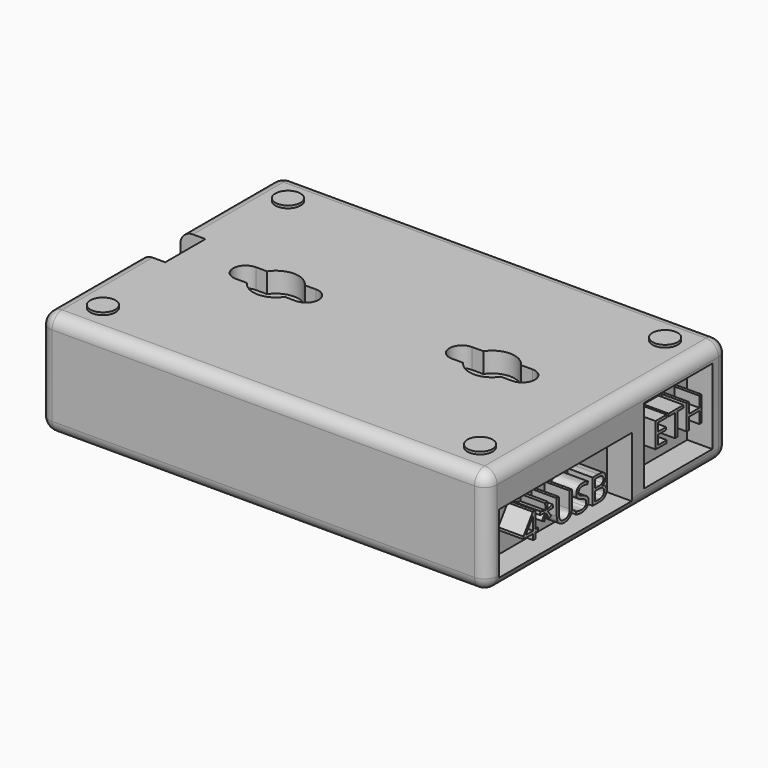
from build123d import *

# Parameters (mm, degrees)
F0_R          = 2.5
F0_W          = 5
F0_H          = 10
F1_DEPTH      = 21
F2_DEPTH      = 0.5
F3_DEPTH      = 4
F4_W          = 17
F4_H          = 15
F4_W_2        = 33
F4_H_2        = 12
F5_DEPTH      = 5
F6_DEPTH      = 5
F7_TEXT_SIZE  = 4.1666666667
F8_DEPTH      = 2
F9_W          = 5.4245442152
F9_H          = 1.6890875995
F9_W_2        = 11.3191977143
F9_H_2        = 3.4400806762
F9_W_3        = 0.1701678839
F9_H_3        = 1.4642129217
F10_DEPTH     = 2
F11_W         = 50
F11_H         = 5
F11_W_2       = 6
F11_H_2       = 22
F12_DEPTH     = 10
F13_T1_DEPTH  = 84
F13_T3_DEPTH  = 55
F13_T5_DEPTH  = 16
F13_T7_DEPTH  = 28.75
F13_T9_DEPTH  = 28.75
F13_S13_W     = 2.5
F13_S13_H     = 2.5
F13_T14_DEPTH = 2.5
F13_S19_W     = 2.5
F13_S19_H     = 2.5
F13_T20_DEPTH = 2.5
F13_S25_W     = 2.5
F13_S25_H     = 2.5
F13_T26_DEPTH = 2.5
F13_S31_W     = 2.5
F13_S31_H     = 2.5
F13_T32_DEPTH = 2.5
F13_S37_W     = 2.5
F13_S37_H     = 2.5
F13_T38_DEPTH = 2.5
F13_S43_W     = 2.5
F13_S43_H     = 2.5
F13_T44_DEPTH = 2.5
F13_S49_W     = 2.5
F13_S49_H     = 2.5
F13_T50_DEPTH = 2.5
F13_S55_W     = 2.5
F13_S55_H     = 2.5
F13_T56_DEPTH = 2.5


# Not quite as in the source:
# - a fillet or chamfer that OpenCascade refuses, or shapes differently, is made with other operations: its cross-section is extruded or revolved along the edge and cut away or added
# - a feature names something its author has since deleted; it is built from what else it names
# - Text() gives the source's letters only with a copy of the font that has no kerning and outlines rounded to 1/6400 em; it was checked with that copy


with BuildPart() as f1:
    # F0 (on Top) → F1 (new body)
    with BuildSketch(Plane.XY):
        Polygon((-44.5, -30), (44.5, -30), (44.5, 30), (-44.5, 30), (-44.5, 5), (-39.5, 5), (-39.5, -5), (-44.5, -5), align=None)
        with Locations((-37.5, -23)):
            Circle(F0_R, mode=Mode.SUBTRACT)
        with Locations((37.5, -23)):
            Circle(F0_R, mode=Mode.SUBTRACT)
        with BuildLine():
            ThreePointArc((-15.5, 2.5), (-13, 0), (-15.5, -2.5))
            Line((-15.5, -2.5), (-17.7583426132, -2.5))
            ThreePointArc((-17.7583426132, -2.5), (-21.5, -4.5), (-25.2416573868, -2.5))
            Line((-25.2416573868, -2.5), (-27.5, -2.5))
            ThreePointArc((-27.5, -2.5), (-30, 0), (-27.5, 2.5))
            Line((-27.5, 2.5), (-25.2416573868, 2.5))
            ThreePointArc((-25.2416573868, 2.5), (-21.5, 4.5), (-17.7583426132, 2.5))
            Line((-17.7583426132, 2.5), (-15.5, 2.5))
        make_face(mode=Mode.SUBTRACT)
        with Locations((-37.5, 23)):
            Circle(F0_R, mode=Mode.SUBTRACT)
        with BuildLine():
            ThreePointArc((25.2416573868, -2.5), (21.5, -4.5), (17.7583426132, -2.5))
            Line((17.7583426132, -2.5), (15.5, -2.5))
            ThreePointArc((15.5, -2.5), (13, 0), (15.5, 2.5))
            Line((15.5, 2.5), (17.7583426132, 2.5))
            ThreePointArc((17.7583426132, 2.5), (21.5, 4.5), (25.2416573868, 2.5))
            Line((25.2416573868, 2.5), (27.5, 2.5))
            ThreePointArc((27.5, 2.5), (30, 0), (27.5, -2.5))
            Line((27.5, -2.5), (25.2416573868, -2.5))
        make_face(mode=Mode.SUBTRACT)
        with Locations((37.5, 23)):
            Circle(F0_R, mode=Mode.SUBTRACT)
        with Locations((-42, 0)):
            Rectangle(F0_W, F0_H)
        with Locations((-37.5, 23)):
            Circle(F0_R)
        with Locations((-37.5, -23)):
            Circle(F0_R)
        with Locations((37.5, 23)):
            Circle(F0_R)
        with Locations((37.5, -23)):
            Circle(F0_R)
        with BuildLine():
            Line((15.5, -2.5), (17.7583426132, -2.5))
            ThreePointArc((17.7583426132, -2.5), (21.5, -4.5), (25.2416573868, -2.5))
            Line((25.2416573868, -2.5), (27.5, -2.5))
            ThreePointArc((27.5, -2.5), (30, 0), (27.5, 2.5))
            Line((27.5, 2.5), (25.2416573868, 2.5))
            ThreePointArc((25.2416573868, 2.5), (21.5, 4.5), (17.7583426132, 2.5))
            Line((17.7583426132, 2.5), (15.5, 2.5))
            ThreePointArc((15.5, 2.5), (13, 0), (15.5, -2.5))
        make_face()
        with BuildLine():
            Line((-17.7583426132, -2.5), (-15.5, -2.5))
            ThreePointArc((-15.5, -2.5), (-13, 0), (-15.5, 2.5))
            Line((-15.5, 2.5), (-17.7583426132, 2.5))
            ThreePointArc((-17.7583426132, 2.5), (-21.5, 4.5), (-25.2416573868, 2.5))
            Line((-25.2416573868, 2.5), (-27.5, 2.5))
            ThreePointArc((-27.5, 2.5), (-30, 0), (-27.5, -2.5))
            Line((-27.5, -2.5), (-25.2416573868, -2.5))
            ThreePointArc((-25.2416573868, -2.5), (-21.5, -4.5), (-17.7583426132, -2.5))
        make_face()
    extrude(amount=-F1_DEPTH)

    # F0 (on Top) → F2 (join)
    with BuildSketch(Plane.XY):
        with Locations((-37.5, 23)):
            Circle(F0_R)
        with Locations((-37.5, -23)):
            Circle(F0_R)
        with Locations((37.5, -23)):
            Circle(F0_R)
        with Locations((37.5, 23)):
            Circle(F0_R)
    extrude(amount=F2_DEPTH)

    # F0 (on Top) → F3 (cut)
    with BuildSketch(Plane.XY):
        with BuildLine():
            Line((15.5, -2.5), (17.7583426132, -2.5))
            ThreePointArc((17.7583426132, -2.5), (21.5, -4.5), (25.2416573868, -2.5))
            Line((25.2416573868, -2.5), (27.5, -2.5))
            ThreePointArc((27.5, -2.5), (30, 0), (27.5, 2.5))
            Line((27.5, 2.5), (25.2416573868, 2.5))
            ThreePointArc((25.2416573868, 2.5), (21.5, 4.5), (17.7583426132, 2.5))
            Line((17.7583426132, 2.5), (15.5, 2.5))
            ThreePointArc((15.5, 2.5), (13, 0), (15.5, -2.5))
        make_face()
        with BuildLine():
            Line((-17.7583426132, -2.5), (-15.5, -2.5))
            ThreePointArc((-15.5, -2.5), (-13, 0), (-15.5, 2.5))
            Line((-15.5, 2.5), (-17.7583426132, 2.5))
            ThreePointArc((-17.7583426132, 2.5), (-21.5, 4.5), (-25.2416573868, 2.5))
            Line((-25.2416573868, 2.5), (-27.5, 2.5))
            ThreePointArc((-27.5, 2.5), (-30, 0), (-27.5, -2.5))
            Line((-27.5, -2.5), (-25.2416573868, -2.5))
            ThreePointArc((-25.2416573868, -2.5), (-21.5, -4.5), (-17.7583426132, -2.5))
        make_face()
    extrude(amount=-F3_DEPTH, mode=Mode.SUBTRACT)

    # F4 (on face) → F5 (cut)
    with BuildSketch(Plane.YZ.offset(44.5)):
        with Locations((17.5, -10.5)):
            Rectangle(F4_W, F4_H)
        Polygon((14.6451822917, -11.7941009895), (14.6451822917, -12.3095089756), (11.8815104167, -12.3095089756), (11.8815104167, -7.3518266839), (14.6451822917, -7.3518266839), (14.6451822917, -7.8639794617), (12.4576822917, -7.8639794617), (12.4576822917, -9.4612016839), (14.5128038194, -9.4612016839), (14.5128038194, -9.9700992534), (12.4576822917, -9.9700992534), (12.4576822917, -11.7941009895), align=None, mode=Mode.SUBTRACT)
        Polygon((17.2688802083, -7.8639794617), (17.2688802083, -12.3095089756), (16.6927083333, -12.3095089756), (16.6927083333, -7.8639794617), (15.1226128472, -7.8639794617), (15.1226128472, -7.3518266839), (18.8389756944, -7.3518266839), (18.8389756944, -7.8639794617), align=None, mode=Mode.SUBTRACT)
        Polygon((23.349609375, -7.3518266839), (23.349609375, -12.3095089756), (22.7734375, -12.3095089756), (22.7734375, -9.97660967), (20.1616753472, -9.97660967), (20.1616753472, -12.3095089756), (19.5855034722, -12.3095089756), (19.5855034722, -7.3518266839), (20.1616753472, -7.3518266839), (20.1616753472, -9.4612016839), (22.7734375, -9.4612016839), (22.7734375, -7.3518266839), align=None, mode=Mode.SUBTRACT)
        with Locations((-10.5, -13)):
            Rectangle(F4_W_2, F4_H_2)
        Polygon((-17.2865668403, -14.1763701994), (-17.2865668403, -14.6885229771), (-18.0222439236, -14.6885229771), (-18.0222439236, -15.8278458938), (-18.5615234375, -15.8278458938), (-18.5615234375, -14.6885229771), (-20.9725477431, -14.6885229771), (-20.9725477431, -14.1969865188), (-18.6190321181, -10.843036866), (-18.0222439236, -10.843036866), (-18.0222439236, -14.1763701994), align=None, mode=Mode.SUBTRACT)
        Polygon((-15.5775824653, -10.5511531855), (-14.9200303819, -10.5511531855), (-15.0654296875, -11.8912139494), (-13.7156032986, -11.5146948521), (-13.6277126736, -12.132099366), (-14.9200303819, -12.2373511021), (-14.0791015625, -13.3419517966), (-14.6617838542, -13.6609622132), (-15.2585720486, -12.4337486716), (-15.8011067708, -13.6609622132), (-16.3978949653, -13.3419517966), (-15.5775824653, -12.2373511021), (-16.8557942708, -12.132099366), (-16.7581380208, -11.5146948521), (-15.4321831597, -11.8912139494), align=None, mode=Mode.SUBTRACT)
        with BuildLine():
            Line((-9.4675564236, -10.8701636021), (-8.8913845486, -10.8701636021))
            Line((-8.8913845486, -10.8701636021), (-8.8913845486, -14.0776288799))
            add(Edge.make_bspline(
                [(-8.8913845486, -14.0776288799), (-8.8913845486, -14.9261531855), (-9.4035373264, -15.4111792271)],
                knots=[0, 0, 0, 1, 1, 1], degree=2))
            add(Edge.make_bspline(
                [(-9.4035373264, -15.4111792271), (-9.9156901042, -15.8962052688), (-10.8108723958, -15.8962052688)],
                knots=[0, 0, 0, 1, 1, 1], degree=2))
            add(Edge.make_bspline(
                [(-10.8108723958, -15.8962052688), (-11.7060546875, -15.8962052688), (-12.1959635417, -15.4073814841)],
                knots=[0, 0, 0, 1, 1, 1], degree=2))
            add(Edge.make_bspline(
                [(-12.1959635417, -15.4073814841), (-12.6858723958, -14.9185576994), (-12.6858723958, -14.0646080466)],
                knots=[0, 0, 0, 1, 1, 1], degree=2))
            Line((-12.6858723958, -14.0646080466), (-12.6858723958, -10.8701636021))
            Line((-12.6858723958, -10.8701636021), (-12.1086154514, -10.8701636021))
            Line((-12.1086154514, -10.8701636021), (-12.1086154514, -14.104755616))
            add(Edge.make_bspline(
                [(-12.1086154514, -14.104755616), (-12.1086154514, -14.7254153382), (-11.76953125, -15.057989123)],
                knots=[0, 0, 0, 1, 1, 1], degree=2))
            add(Edge.make_bspline(
                [(-11.76953125, -15.057989123), (-11.4304470486, -15.3905629077), (-10.7728949653, -15.3905629077)],
                knots=[0, 0, 0, 1, 1, 1], degree=2))
            add(Edge.make_bspline(
                [(-10.7728949653, -15.3905629077), (-10.1457248264, -15.3905629077), (-9.806640625, -15.0563615188)],
                knots=[0, 0, 0, 1, 1, 1], degree=2))
            add(Edge.make_bspline(
                [(-9.806640625, -15.0563615188), (-9.4675564236, -14.7221601299), (-9.4675564236, -14.0982451994)],
                knots=[0, 0, 0, 1, 1, 1], degree=2))
            Line((-9.4675564236, -14.0982451994), (-9.4675564236, -10.8701636021))
        make_face(mode=Mode.SUBTRACT)
        with BuildLine():
            add(Edge.make_bspline(
                [(-5.0751953125, -13.6815785327), (-4.7822265625, -14.0005889494), (-4.7822265625, -14.5084014494)],
                knots=[0, 0, 0, 1, 1, 1], degree=2))
            add(Edge.make_bspline(
                [(-4.7822265625, -14.5084014494), (-4.7822265625, -15.1626983244), (-5.2569444444, -15.5294517966)],
                knots=[0, 0, 0, 1, 1, 1], degree=2))
            add(Edge.make_bspline(
                [(-5.2569444444, -15.5294517966), (-5.7316623264, -15.8962052688), (-6.5454644097, -15.8962052688)],
                knots=[0, 0, 0, 1, 1, 1], degree=2))
            add(Edge.make_bspline(
                [(-6.5454644097, -15.8962052688), (-7.4265407986, -15.8962052688), (-7.9018012153, -15.6683406855)],
                knots=[0, 0, 0, 1, 1, 1], degree=2))
            Line((-7.9018012153, -15.6683406855), (-7.9018012153, -15.1127851299))
            add(Edge.make_bspline(
                [(-7.9018012153, -15.1127851299), (-7.5958116319, -15.2408233244), (-7.2366536458, -15.315693116)],
                knots=[0, 0, 0, 1, 1, 1], degree=2))
            add(Edge.make_bspline(
                [(-7.2366536458, -15.315693116), (-6.8774956597, -15.3905629077), (-6.5248480903, -15.3905629077)],
                knots=[0, 0, 0, 1, 1, 1], degree=2))
            add(Edge.make_bspline(
                [(-6.5248480903, -15.3905629077), (-5.9486762153, -15.3905629077), (-5.6567925347, -15.1719214146)],
                knots=[0, 0, 0, 1, 1, 1], degree=2))
            add(Edge.make_bspline(
                [(-5.6567925347, -15.1719214146), (-5.3649088542, -14.9532799216), (-5.3649088542, -14.5626549216)],
                knots=[0, 0, 0, 1, 1, 1], degree=2))
            add(Edge.make_bspline(
                [(-5.3649088542, -14.5626549216), (-5.3649088542, -14.3054934632), (-5.4685329861, -14.1411054424)],
                knots=[0, 0, 0, 1, 1, 1], degree=2))
            add(Edge.make_bspline(
                [(-5.4685329861, -14.1411054424), (-5.5721571181, -13.9767174216), (-5.8146701389, -13.837285998)],
                knots=[0, 0, 0, 1, 1, 1], degree=2))
            add(Edge.make_bspline(
                [(-5.8146701389, -13.837285998), (-6.0571831597, -13.6978545744), (-6.5519748264, -13.5220733244)],
                knots=[0, 0, 0, 1, 1, 1], degree=2))
            add(Edge.make_bspline(
                [(-6.5519748264, -13.5220733244), (-7.2431640625, -13.274677491), (-7.5399305556, -12.9355932896)],
                knots=[0, 0, 0, 1, 1, 1], degree=2))
            add(Edge.make_bspline(
                [(-7.5399305556, -12.9355932896), (-7.8366970486, -12.5965090882), (-7.8366970486, -12.0507191577)],
                knots=[0, 0, 0, 1, 1, 1], degree=2))
            add(Edge.make_bspline(
                [(-7.8366970486, -12.0507191577), (-7.8366970486, -11.477802491), (-7.4064670139, -11.1387182896)],
                knots=[0, 0, 0, 1, 1, 1], degree=2))
            add(Edge.make_bspline(
                [(-7.4064670139, -11.1387182896), (-6.9762369792, -10.7996340882), (-6.2666015625, -10.7996340882)],
                knots=[0, 0, 0, 1, 1, 1], degree=2))
            add(Edge.make_bspline(
                [(-6.2666015625, -10.7996340882), (-5.5276692708, -10.7996340882), (-4.9070095486, -11.0709014494)],
                knots=[0, 0, 0, 1, 1, 1], degree=2))
            Line((-4.9070095486, -11.0709014494), (-5.0871310764, -11.5722035327))
            add(Edge.make_bspline(
                [(-5.0871310764, -11.5722035327), (-5.7012803819, -11.3150420744), (-6.2807074653, -11.3150420744)],
                knots=[0, 0, 0, 1, 1, 1], degree=2))
            add(Edge.make_bspline(
                [(-6.2807074653, -11.3150420744), (-6.7386067708, -11.3150420744), (-6.9963107639, -11.5114396438)],
                knots=[0, 0, 0, 1, 1, 1], degree=2))
            add(Edge.make_bspline(
                [(-6.9963107639, -11.5114396438), (-7.2540147569, -11.7078372132), (-7.2540147569, -12.0572295744)],
                knots=[0, 0, 0, 1, 1, 1], degree=2))
            add(Edge.make_bspline(
                [(-7.2540147569, -12.0572295744), (-7.2540147569, -12.3143910327), (-7.1590711806, -12.4793215882)],
                knots=[0, 0, 0, 1, 1, 1], degree=2))
            add(Edge.make_bspline(
                [(-7.1590711806, -12.4793215882), (-7.0641276042, -12.6442521438), (-6.8384331597, -12.7815134285)],
                knots=[0, 0, 0, 1, 1, 1], degree=2))
            add(Edge.make_bspline(
                [(-6.8384331597, -12.7815134285), (-6.6127387153, -12.9187747132), (-6.1483289931, -13.0847903382)],
                knots=[0, 0, 0, 1, 1, 1], degree=2))
            add(Edge.make_bspline(
                [(-6.1483289931, -13.0847903382), (-5.3681640625, -13.362568116), (-5.0751953125, -13.6815785327)],
                knots=[0, 0, 0, 1, 1, 1], degree=2))
        make_face(mode=Mode.SUBTRACT)
        with BuildLine():
            Line((-3.7676866319, -15.8278458938), (-3.7676866319, -10.8701636021))
            Line((-3.7676866319, -10.8701636021), (-2.3668619792, -10.8701636021))
            add(Edge.make_bspline(
                [(-2.3668619792, -10.8701636021), (-1.3805338542, -10.8701636021), (-0.939453125, -11.165302491)],
                knots=[0, 0, 0, 1, 1, 1], degree=2))
            add(Edge.make_bspline(
                [(-0.939453125, -11.165302491), (-0.4983723958, -11.4604413799), (-0.4983723958, -12.0973771438)],
                knots=[0, 0, 0, 1, 1, 1], degree=2))
            add(Edge.make_bspline(
                [(-0.4983723958, -12.0973771438), (-0.4983723958, -12.5390004077), (-0.744140625, -12.825458741)],
                knots=[0, 0, 0, 1, 1, 1], degree=2))
            add(Edge.make_bspline(
                [(-0.744140625, -12.825458741), (-0.9899088542, -13.1119170744), (-1.4619140625, -13.196552491)],
                knots=[0, 0, 0, 1, 1, 1], degree=2))
            Line((-1.4619140625, -13.196552491), (-1.4619140625, -13.2301896438))
            add(Edge.make_bspline(
                [(-1.4619140625, -13.2301896438), (-0.3323567708, -13.4233320049), (-0.3323567708, -14.417255616)],
                knots=[0, 0, 0, 1, 1, 1], degree=2))
            add(Edge.make_bspline(
                [(-0.3323567708, -14.417255616), (-0.3323567708, -15.081318116), (-0.7815755208, -15.4545820049)],
                knots=[0, 0, 0, 1, 1, 1], degree=2))
            add(Edge.make_bspline(
                [(-0.7815755208, -15.4545820049), (-1.2307942708, -15.8278458938), (-2.0380859375, -15.8278458938)],
                knots=[0, 0, 0, 1, 1, 1], degree=2))
            Line((-2.0380859375, -15.8278458938), (-3.7676866319, -15.8278458938))
        make_face(mode=Mode.SUBTRACT)
        with BuildLine():
            Line((-3.1915147569, -11.3692955466), (-3.1915147569, -12.9925594355))
            Line((-3.1915147569, -12.9925594355), (-2.2420789931, -12.9925594355))
            add(Edge.make_bspline(
                [(-2.2420789931, -12.9925594355), (-1.6311848958, -12.9925594355), (-1.3631727431, -12.8010446785)],
                knots=[0, 0, 0, 1, 1, 1], degree=2))
            add(Edge.make_bspline(
                [(-1.3631727431, -12.8010446785), (-1.0951605903, -12.6095299216), (-1.0951605903, -12.1559708938)],
                knots=[0, 0, 0, 1, 1, 1], degree=2))
            add(Edge.make_bspline(
                [(-1.0951605903, -12.1559708938), (-1.0951605903, -11.7382191577), (-1.3935546875, -11.5537573521)],
                knots=[0, 0, 0, 1, 1, 1], degree=2))
            add(Edge.make_bspline(
                [(-1.3935546875, -11.5537573521), (-1.6919487847, -11.3692955466), (-2.3429904514, -11.3692955466)],
                knots=[0, 0, 0, 1, 1, 1], degree=2))
            Line((-2.3429904514, -11.3692955466), (-3.1915147569, -11.3692955466))
        make_face()
        with BuildLine():
            Line((-2.2041015625, -13.4808406855), (-3.1915147569, -13.4808406855))
            Line((-3.1915147569, -13.4808406855), (-3.1915147569, -15.3363094355))
            Line((-3.1915147569, -15.3363094355), (-2.1563585069, -15.3363094355))
            add(Edge.make_bspline(
                [(-2.1563585069, -15.3363094355), (-1.5563151042, -15.3363094355), (-1.2530381944, -15.1041045744)],
                knots=[0, 0, 0, 1, 1, 1], degree=2))
            add(Edge.make_bspline(
                [(-1.2530381944, -15.1041045744), (-0.9497612847, -14.8718997132), (-0.9497612847, -14.3760229771)],
                knots=[0, 0, 0, 1, 1, 1], degree=2))
            add(Edge.make_bspline(
                [(-0.9497612847, -14.3760229771), (-0.9497612847, -13.9148684632), (-1.2600911458, -13.6978545744)],
                knots=[0, 0, 0, 1, 1, 1], degree=2))
            add(Edge.make_bspline(
                [(-1.2600911458, -13.6978545744), (-1.5704210069, -13.4808406855), (-2.2041015625, -13.4808406855)],
                knots=[0, 0, 0, 1, 1, 1], degree=2))
        make_face()
        with BuildLine():
            Line((-20.4093967014, -14.1763701994), (-18.5615234375, -14.1763701994))
            Line((-18.5615234375, -14.1763701994), (-18.5615234375, -12.5281497132))
            add(Edge.make_bspline(
                [(-18.5615234375, -12.5281497132), (-18.5615234375, -12.0431236716), (-18.5268012153, -11.4333146438)],
                knots=[0, 0, 0, 1, 1, 1], degree=2))
            Line((-18.5268012153, -11.4333146438), (-18.5539279514, -11.4333146438))
            add(Edge.make_bspline(
                [(-18.5539279514, -11.4333146438), (-18.7166883681, -11.7588354771), (-18.8599175347, -11.9725941577)],
                knots=[0, 0, 0, 1, 1, 1], degree=2))
            Line((-18.8599175347, -11.9725941577), (-20.4093967014, -14.1763701994))
        make_face()
    extrude(amount=-F5_DEPTH, mode=Mode.SUBTRACT)

    # F0 (on Top) → F6 (cut)
    with BuildSketch(Plane.XY):
        with Locations((-42, 0)):
            Rectangle(F0_W, F0_H)
    extrude(amount=-F6_DEPTH, mode=Mode.SUBTRACT)

    # F7 (on face) → F8 (cut)
    with BuildSketch(Plane.XY.offset(-5)):
        with Locations(Location((-40.6651311529, -2.6702473958), (0, 0, 90))):
            Text('SD', F7_TEXT_SIZE, font='Open Sans', text_align=(TextAlign.LEFT, TextAlign.BOTTOM))
    extrude(amount=-F8_DEPTH, mode=Mode.SUBTRACT)

    # F9 (on face) → F10 (cut)
    with BuildSketch(Plane(origin=(0, 30, 0), x_dir=(-1, 0, 0), z_dir=(0, 1, 0))):
        with Locations((35.1204499602, -5.5329566821)):
            Rectangle(F9_W, F9_H)
        with BuildLine():
            Line((35.1204437552, -5.1798889881), (35.1917698958, -5.1798889881))
            Line((35.1917698958, -5.1798889881), (35.1917698958, -5.5769512701))
            add(Edge.make_bspline(
                [(35.1917698958, -5.5769512701), (35.1917698958, -5.6819927804), (35.1283688819, -5.7420356898)],
                knots=[0, 0, 0, 1, 1, 1], degree=2))
            add(Edge.make_bspline(
                [(35.1283688819, -5.7420356898), (35.064967868, -5.8020785991), (34.9541504179, -5.8020785991)],
                knots=[0, 0, 0, 1, 1, 1], degree=2))
            add(Edge.make_bspline(
                [(34.9541504179, -5.8020785991), (34.8433329677, -5.8020785991), (34.7826855996, -5.7415655551)],
                knots=[0, 0, 0, 1, 1, 1], degree=2))
            add(Edge.make_bspline(
                [(34.7826855996, -5.7415655551), (34.7220382314, -5.6810525111), (34.7220382314, -5.5753393799)],
                knots=[0, 0, 0, 1, 1, 1], degree=2))
            Line((34.7220382314, -5.5753393799), (34.7220382314, -5.1798889881))
            Line((34.7220382314, -5.1798889881), (34.7934986962, -5.1798889881))
            Line((34.7934986962, -5.1798889881), (34.7934986962, -5.5803093746))
            add(Edge.make_bspline(
                [(34.7934986962, -5.5803093746), (34.7934986962, -5.6571428067), (34.8354750031, -5.6983131685)],
                knots=[0, 0, 0, 1, 1, 1], degree=2))
            add(Edge.make_bspline(
                [(34.8354750031, -5.6983131685), (34.87745131, -5.7394835303), (34.9588517643, -5.7394835303)],
                knots=[0, 0, 0, 1, 1, 1], degree=2))
            add(Edge.make_bspline(
                [(34.9588517643, -5.7394835303), (35.0364911415, -5.7394835303), (35.0784674483, -5.6981116822)],
                knots=[0, 0, 0, 1, 1, 1], degree=2))
            add(Edge.make_bspline(
                [(35.0784674483, -5.6981116822), (35.1204437552, -5.6567398342), (35.1204437552, -5.5795034295)],
                knots=[0, 0, 0, 1, 1, 1], degree=2))
            Line((35.1204437552, -5.5795034295), (35.1204437552, -5.1798889881))
        make_face(mode=Mode.SUBTRACT)
        with BuildLine():
            add(Edge.make_bspline(
                [(35.6641880439, -5.5279229437), (35.7004555731, -5.5674142532), (35.7004555731, -5.6302779703)],
                knots=[0, 0, 0, 1, 1, 1], degree=2))
            add(Edge.make_bspline(
                [(35.7004555731, -5.6302779703), (35.7004555731, -5.7112754521), (35.6416887435, -5.7566770256)],
                knots=[0, 0, 0, 1, 1, 1], degree=2))
            add(Edge.make_bspline(
                [(35.6416887435, -5.7566770256), (35.5829219138, -5.8020785991), (35.4821787773, -5.8020785991)],
                knots=[0, 0, 0, 1, 1, 1], degree=2))
            add(Edge.make_bspline(
                [(35.4821787773, -5.8020785991), (35.3731075415, -5.8020785991), (35.3142735498, -5.7738705209)],
                knots=[0, 0, 0, 1, 1, 1], degree=2))
            Line((35.3142735498, -5.7738705209), (35.3142735498, -5.7050965397))
            add(Edge.make_bspline(
                [(35.3142735498, -5.7050965397), (35.3521529692, -5.7209467932), (35.3966142734, -5.7302151617)],
                knots=[0, 0, 0, 1, 1, 1], degree=2))
            add(Edge.make_bspline(
                [(35.3966142734, -5.7302151617), (35.4410755776, -5.7394835303), (35.4847309368, -5.7394835303)],
                knots=[0, 0, 0, 1, 1, 1], degree=2))
            add(Edge.make_bspline(
                [(35.4847309368, -5.7394835303), (35.5560570774, -5.7394835303), (35.5921902824, -5.7124172076)],
                knots=[0, 0, 0, 1, 1, 1], degree=2))
            add(Edge.make_bspline(
                [(35.5921902824, -5.7124172076), (35.6283234873, -5.685350885), (35.6283234873, -5.6369941794)],
                knots=[0, 0, 0, 1, 1, 1], degree=2))
            add(Edge.make_bspline(
                [(35.6283234873, -5.6369941794), (35.6283234873, -5.6051593483), (35.615495528, -5.5848092347)],
                knots=[0, 0, 0, 1, 1, 1], degree=2))
            add(Edge.make_bspline(
                [(35.615495528, -5.5848092347), (35.6026675686, -5.5644591212), (35.5726461139, -5.5471984638)],
                knots=[0, 0, 0, 1, 1, 1], degree=2))
            add(Edge.make_bspline(
                [(35.5726461139, -5.5471984638), (35.5426246592, -5.5299378064), (35.4813728322, -5.5081772889)],
                knots=[0, 0, 0, 1, 1, 1], degree=2))
            add(Edge.make_bspline(
                [(35.4813728322, -5.5081772889), (35.3958083283, -5.4775513754), (35.3590706645, -5.4355750685)],
                knots=[0, 0, 0, 1, 1, 1], degree=2))
            add(Edge.make_bspline(
                [(35.3590706645, -5.4355750685), (35.3223330007, -5.3935987617), (35.3223330007, -5.3260336981)],
                knots=[0, 0, 0, 1, 1, 1], degree=2))
            add(Edge.make_bspline(
                [(35.3223330007, -5.3260336981), (35.3223330007, -5.25511053), (35.3755925389, -5.2131342231)],
                knots=[0, 0, 0, 1, 1, 1], degree=2))
            add(Edge.make_bspline(
                [(35.3755925389, -5.2131342231), (35.4288520771, -5.1711579163), (35.5167000921, -5.1711579163)],
                knots=[0, 0, 0, 1, 1, 1], degree=2))
            add(Edge.make_bspline(
                [(35.5167000921, -5.1711579163), (35.60817486, -5.1711579163), (35.6850082921, -5.2047389618)],
                knots=[0, 0, 0, 1, 1, 1], degree=2))
            Line((35.6850082921, -5.2047389618), (35.6627104779, -5.2667967338))
            add(Edge.make_bspline(
                [(35.6627104779, -5.2667967338), (35.5866829909, -5.2349619027), (35.5149538777, -5.2349619027)],
                knots=[0, 0, 0, 1, 1, 1], degree=2))
            add(Edge.make_bspline(
                [(35.5149538777, -5.2349619027), (35.4582690729, -5.2349619027), (35.4263670797, -5.2592745797)],
                knots=[0, 0, 0, 1, 1, 1], degree=2))
            add(Edge.make_bspline(
                [(35.4263670797, -5.2592745797), (35.3944650865, -5.2835872566), (35.3944650865, -5.3268396432)],
                knots=[0, 0, 0, 1, 1, 1], degree=2))
            add(Edge.make_bspline(
                [(35.3944650865, -5.3268396432), (35.3944650865, -5.3586744743), (35.4062184524, -5.37909175)],
                knots=[0, 0, 0, 1, 1, 1], degree=2))
            add(Edge.make_bspline(
                [(35.4062184524, -5.37909175), (35.4179718183, -5.3995090257), (35.4459112482, -5.4165010347)],
                knots=[0, 0, 0, 1, 1, 1], degree=2))
            add(Edge.make_bspline(
                [(35.4459112482, -5.4165010347), (35.473850678, -5.4334930437), (35.5313414279, -5.4540446436)],
                knots=[0, 0, 0, 1, 1, 1], degree=2))
            add(Edge.make_bspline(
                [(35.5313414279, -5.4540446436), (35.6279205148, -5.4884316341), (35.6641880439, -5.5279229437)],
                knots=[0, 0, 0, 1, 1, 1], degree=2))
        make_face(mode=Mode.SUBTRACT)
        with BuildLine():
            Line((35.8260486832, -5.7936161757), (35.8260486832, -5.1798889881))
            Line((35.8260486832, -5.1798889881), (35.9994612022, -5.1798889881))
            add(Edge.make_bspline(
                [(35.9994612022, -5.1798889881), (36.1215618836, -5.1798889881), (36.1761646636, -5.2164251656)],
                knots=[0, 0, 0, 1, 1, 1], degree=2))
            add(Edge.make_bspline(
                [(36.1761646636, -5.2164251656), (36.2307674436, -5.2529613431), (36.2307674436, -5.3318096379)],
                knots=[0, 0, 0, 1, 1, 1], degree=2))
            add(Edge.make_bspline(
                [(36.2307674436, -5.3318096379), (36.2307674436, -5.38647958), (36.2003430164, -5.4219411641)],
                knots=[0, 0, 0, 1, 1, 1], degree=2))
            add(Edge.make_bspline(
                [(36.2003430164, -5.4219411641), (36.1699185892, -5.4574027481), (36.11148757, -5.4678800343)],
                knots=[0, 0, 0, 1, 1, 1], degree=2))
            Line((36.11148757, -5.4678800343), (36.11148757, -5.4720440839))
            add(Edge.make_bspline(
                [(36.11148757, -5.4720440839), (36.2513190435, -5.4959537883), (36.2513190435, -5.6189947391)],
                knots=[0, 0, 0, 1, 1, 1], degree=2))
            add(Edge.make_bspline(
                [(36.2513190435, -5.6189947391), (36.2513190435, -5.7012011384), (36.1957088321, -5.747408657)],
                knots=[0, 0, 0, 1, 1, 1], degree=2))
            add(Edge.make_bspline(
                [(36.1957088321, -5.747408657), (36.1400986208, -5.7936161757), (36.0401614294, -5.7936161757)],
                knots=[0, 0, 0, 1, 1, 1], degree=2))
            Line((36.0401614294, -5.7936161757), (35.8260486832, -5.7936161757))
        make_face(mode=Mode.SUBTRACT)
        with Locations((24.0754019469, -7.6189141255)):
            Rectangle(F9_W_2, F9_H_2)
        Polygon((22.7060472052, -6.7842903982), (22.7060472052, -8.2485033199), (22.5358793214, -8.2485033199), (22.5358793214, -7.559499647), (21.7645156745, -7.559499647), (21.7645156745, -8.2485033199), (21.5943477906, -8.2485033199), (21.5943477906, -6.7842903982), (21.7645156745, -6.7842903982), (21.7645156745, -7.4072779053), (22.5358793214, -7.4072779053), (22.5358793214, -6.7842903982), align=None, mode=Mode.SUBTRACT)
        with BuildLine():
            add(Edge.make_bspline(
                [(24.087098986, -6.9735260581), (24.2763346459, -7.1627617181), (24.2763346459, -7.5024565522)],
                knots=[0, 0, 0, 1, 1, 1], degree=2))
            add(Edge.make_bspline(
                [(24.2763346459, -7.5024565522), (24.2763346459, -7.8649045308), (24.0795680156, -8.0567039254)],
                knots=[0, 0, 0, 1, 1, 1], degree=2))
            add(Edge.make_bspline(
                [(24.0795680156, -8.0567039254), (23.8828013853, -8.2485033199), (23.5133031365, -8.2485033199)],
                knots=[0, 0, 0, 1, 1, 1], degree=2))
            Line((23.5133031365, -8.2485033199), (23.1075921365, -8.2485033199))
            Line((23.1075921365, -8.2485033199), (23.1075921365, -6.7842903982))
            Line((23.1075921365, -6.7842903982), (23.556245691, -6.7842903982))
            add(Edge.make_bspline(
                [(23.556245691, -6.7842903982), (23.8978633261, -6.7842903982), (24.087098986, -6.9735260581)],
                knots=[0, 0, 0, 1, 1, 1], degree=2))
        make_face(mode=Mode.SUBTRACT)
        with BuildLine():
            Line((25.3880340606, -8.2485033199), (25.2508742597, -8.2485033199))
            Line((25.2508742597, -8.2485033199), (24.7541506815, -6.9506126802))
            Line((24.7541506815, -6.9506126802), (24.7461390109, -6.9506126802))
            add(Edge.make_bspline(
                [(24.7461390109, -6.9506126802), (24.7602395511, -7.1047572228), (24.7602395511, -7.3172267275)],
                knots=[0, 0, 0, 1, 1, 1], degree=2))
            Line((24.7602395511, -7.3172267275), (24.7602395511, -8.2485033199))
            Line((24.7602395511, -8.2485033199), (24.6028903402, -8.2485033199))
            Line((24.6028903402, -8.2485033199), (24.6028903402, -6.7842903982))
            Line((24.6028903402, -6.7842903982), (24.8592638, -6.7842903982))
            Line((24.8592638, -6.7842903982), (25.3229792952, -7.9921298602))
            Line((25.3229792952, -7.9921298602), (25.3309909658, -7.9921298602))
            Line((25.3309909658, -7.9921298602), (25.798552063, -6.7842903982))
            Line((25.798552063, -6.7842903982), (26.0530027217, -6.7842903982))
            Line((26.0530027217, -6.7842903982), (26.0530027217, -8.2485033199))
            Line((26.0530027217, -8.2485033199), (25.8828348378, -8.2485033199))
            Line((25.8828348378, -8.2485033199), (25.8828348378, -7.3050489882))
            add(Edge.make_bspline(
                [(25.8828348378, -7.3050489882), (25.8828348378, -7.1428927749), (25.8969353781, -6.9525354811)],
                knots=[0, 0, 0, 1, 1, 1], degree=2))
            Line((25.8969353781, -6.9525354811), (25.8889237075, -6.9525354811))
            Line((25.8889237075, -6.9525354811), (25.3880340606, -8.2485033199))
        make_face(mode=Mode.SUBTRACT)
        with Locations((26.5396315949, -7.516396859)):
            Rectangle(F9_W_3, F9_H_3, mode=Mode.SUBTRACT)
        with BuildLine():
            add(Edge.make_bspline(
                [(23.9428889149, -7.9515908069), (24.0962322905, -7.8017725664), (24.0962322905, -7.5085454218)],
                knots=[0, 0, 0, 1, 1, 1], degree=2))
            add(Edge.make_bspline(
                [(24.0962322905, -7.5085454218), (24.0962322905, -7.2220480806), (23.9525029197, -7.0768766091)],
                knots=[0, 0, 0, 1, 1, 1], degree=2))
            add(Edge.make_bspline(
                [(23.9525029197, -7.0768766091), (23.8087735488, -6.9317051375), (23.525160409, -6.9317051375)],
                knots=[0, 0, 0, 1, 1, 1], degree=2))
            Line((23.525160409, -6.9317051375), (23.2777600204, -6.9317051375))
            Line((23.2777600204, -6.9317051375), (23.2777600204, -8.1014090474))
            Line((23.2777600204, -8.1014090474), (23.4851020559, -8.1014090474))
            add(Edge.make_bspline(
                [(23.4851020559, -8.1014090474), (23.7895455393, -8.1014090474), (23.9428889149, -7.9515908069)],
                knots=[0, 0, 0, 1, 1, 1], degree=2))
        make_face()
        with BuildLine():
            Line((35.8973748239, -5.2416781118), (35.8973748239, -5.4426270881))
            Line((35.8973748239, -5.4426270881), (36.0149084831, -5.4426270881))
            add(Edge.make_bspline(
                [(36.0149084831, -5.4426270881), (36.0905329976, -5.4426270881), (36.1237110706, -5.41891887)],
                knots=[0, 0, 0, 1, 1, 1], degree=2))
            add(Edge.make_bspline(
                [(36.1237110706, -5.41891887), (36.1568891435, -5.3952106518), (36.1568891435, -5.3390631438)],
                knots=[0, 0, 0, 1, 1, 1], degree=2))
            add(Edge.make_bspline(
                [(36.1568891435, -5.3390631438), (36.1568891435, -5.2873483337), (36.1199499935, -5.2645132228)],
                knots=[0, 0, 0, 1, 1, 1], degree=2))
            add(Edge.make_bspline(
                [(36.1199499935, -5.2645132228), (36.0830108434, -5.2416781118), (36.0024163342, -5.2416781118)],
                knots=[0, 0, 0, 1, 1, 1], degree=2))
            Line((36.0024163342, -5.2416781118), (35.8973748239, -5.2416781118))
        make_face()
        with BuildLine():
            Line((36.0196098295, -5.50307297), (35.8973748239, -5.50307297))
            Line((35.8973748239, -5.50307297), (35.8973748239, -5.7327673212))
            Line((35.8973748239, -5.7327673212), (36.0255200935, -5.7327673212))
            add(Edge.make_bspline(
                [(36.0255200935, -5.7327673212), (36.0998013662, -5.7327673212), (36.137344975, -5.7040219463)],
                knots=[0, 0, 0, 1, 1, 1], degree=2))
            add(Edge.make_bspline(
                [(36.137344975, -5.7040219463), (36.1748885839, -5.6752765713), (36.1748885839, -5.6138904201)],
                knots=[0, 0, 0, 1, 1, 1], degree=2))
            add(Edge.make_bspline(
                [(36.1748885839, -5.6138904201), (36.1748885839, -5.5568026428), (36.1364718678, -5.5299378064)],
                knots=[0, 0, 0, 1, 1, 1], degree=2))
            add(Edge.make_bspline(
                [(36.1364718678, -5.5299378064), (36.0980551518, -5.50307297), (36.0196098295, -5.50307297)],
                knots=[0, 0, 0, 1, 1, 1], degree=2))
        make_face()
    extrude(amount=-F10_DEPTH, mode=Mode.SUBTRACT)

    # F11 (on face) → F12 (cut)
    with BuildSketch(Plane(origin=(0, 0, -21), x_dir=(1, 0, 0), z_dir=(0, 0, -1))):
        with Locations((-14.5, 23.5)):
            Rectangle(F11_W, F11_H)
        with Locations((3.5, -16)):
            Rectangle(F11_W_2, F11_H_2)
    extrude(amount=-F12_DEPTH, mode=Mode.SUBTRACT)

    # F13: fillet of radius 2.5 on 13 edges, made by hand

    # F13_s2 → F13_t1 (cut)
    with BuildSketch(Plane.YZ.offset(-42)):
        with BuildLine():
            ThreePointArc((-30, -18.5), (-29.267766953, -20.267766953), (-27.5, -21))
            Line((-27.5, -21), (-30, -21))
            Line((-30, -21), (-30, -18.5))
        make_face()
        with BuildLine():
            ThreePointArc((27.5, -21), (29.267766953, -20.267766953), (30, -18.5))
            Line((30, -18.5), (30, -21))
            Line((30, -21), (27.5, -21))
        make_face()
        with BuildLine():
            ThreePointArc((-30, -2.5), (-29.267766953, -0.732233047), (-27.5, 0))
            Line((-27.5, 0), (-30, 0))
            Line((-30, 0), (-30, -2.5))
        make_face()
        with BuildLine():
            ThreePointArc((27.5, 0), (29.267766953, -0.732233047), (30, -2.5))
            Line((30, -2.5), (30, 0))
            Line((30, 0), (27.5, 0))
        make_face()
    extrude(amount=F13_T1_DEPTH, mode=Mode.SUBTRACT)

    # F13_s4 → F13_t3 (cut)
    with BuildSketch(Plane.XZ.offset(-27.5)):
        with BuildLine():
            ThreePointArc((-44.5, -18.5), (-43.767766953, -20.267766953), (-42, -21))
            Line((-42, -21), (-44.5, -21))
            Line((-44.5, -21), (-44.5, -18.5))
        make_face()
        with BuildLine():
            ThreePointArc((44.5, -18.5), (43.767766953, -20.267766953), (42, -21))
            Line((42, -21), (44.5, -21))
            Line((44.5, -21), (44.5, -18.5))
        make_face()
        with BuildLine():
            ThreePointArc((44.5, -2.5), (43.767766953, -0.732233047), (42, 0))
            Line((42, 0), (44.5, 0))
            Line((44.5, 0), (44.5, -2.5))
        make_face()
    extrude(amount=F13_T3_DEPTH, mode=Mode.SUBTRACT)

    # F13_s6 → F13_t5 (cut)
    with BuildSketch(Plane.XY.offset(-18.5)):
        with BuildLine():
            ThreePointArc((-44.5, 27.5), (-43.767766953, 29.267766953), (-42, 30))
            Line((-42, 30), (-44.5, 30))
            Line((-44.5, 30), (-44.5, 27.5))
        make_face()
        with BuildLine():
            ThreePointArc((44.5, 27.5), (43.767766953, 29.267766953), (42, 30))
            Line((42, 30), (44.5, 30))
            Line((44.5, 30), (44.5, 27.5))
        make_face()
        with BuildLine():
            ThreePointArc((42, -30), (43.767766953, -29.267766953), (44.5, -27.5))
            Line((44.5, -27.5), (44.5, -30))
            Line((44.5, -30), (42, -30))
        make_face()
        with BuildLine():
            ThreePointArc((-42, -30), (-43.767766953, -29.267766953), (-44.5, -27.5))
            Line((-44.5, -27.5), (-44.5, -30))
            Line((-44.5, -30), (-42, -30))
        make_face()
    extrude(amount=F13_T5_DEPTH, mode=Mode.SUBTRACT)

    # F13_s8 → F13_t7 (cut)
    with BuildSketch(Plane.XZ.offset(-27.5)):
        with BuildLine():
            ThreePointArc((-44.5, -2.5), (-43.767766953, -0.732233047), (-42, 0))
            Line((-42, 0), (-44.5, 0))
            Line((-44.5, 0), (-44.5, -2.5))
        make_face()
    extrude(amount=F13_T7_DEPTH, mode=Mode.SUBTRACT)

    # F13_s10 → F13_t9 (cut)
    with BuildSketch(Plane.XZ.offset(-1.25)):
        with BuildLine():
            ThreePointArc((-44.5, -2.5), (-43.767766953, -0.732233047), (-42, 0))
            Line((-42, 0), (-44.5, 0))
            Line((-44.5, 0), (-44.5, -2.5))
        make_face()
    extrude(amount=F13_T9_DEPTH, mode=Mode.SUBTRACT)


with BuildPart() as f13_tool12:
    # F13_s13 → F13_t14 (new body)
    with BuildSketch(Plane.XZ.offset(27.5)):
        with Locations((-43.25, -19.75)):
            Rectangle(F13_S13_W, F13_S13_H)
    extrude(amount=F13_T14_DEPTH)

    # F13_s15 → F13_t16 (revolve, cut)
    with BuildSketch(Plane(origin=(-42, -27.5, -18.5), x_dir=(0.7071067812, 0, 0.7071067812), z_dir=(0.7071067812, 0, -0.7071067812))):
        with BuildLine():
            ThreePointArc((0, -2.5), (2.5, 0), (0, 2.5))
            Line((0, 2.5), (0, -2.5))
        make_face()
    revolve(axis=Axis((-42, -27.5, -18.5), (0, -1, 0)), mode=Mode.SUBTRACT)


with BuildPart() as f1_1:
    add(f1.part)

    # F13_t11: cut F13_tool12
    add(f13_tool12.part, mode=Mode.SUBTRACT)


with BuildPart() as f13_tool18:
    # F13_s19 → F13_t20 (new body)
    with BuildSketch(Plane.XZ.offset(27.5)):
        with Locations((43.25, -19.75)):
            Rectangle(F13_S19_W, F13_S19_H)
    extrude(amount=F13_T20_DEPTH)

    # F13_s21 → F13_t22 (revolve, cut)
    with BuildSketch(Plane(origin=(42, -27.5, -18.5), x_dir=(-0.7071067812, 0, 0.7071067812), z_dir=(0.7071067812, 0, 0.7071067812))):
        with BuildLine():
            ThreePointArc((0, -2.5), (2.5, 0), (0, 2.5))
            Line((0, 2.5), (0, -2.5))
        make_face()
    revolve(axis=Axis((42, -27.5, -18.5), (0, -1, 0)), mode=Mode.SUBTRACT)


with BuildPart() as f1_2:
    add(f1_1.part)

    # F13_t17: cut F13_tool18
    add(f13_tool18.part, mode=Mode.SUBTRACT)


with BuildPart() as f13_tool24:
    # F13_s25 → F13_t26 (new body)
    with BuildSketch(Plane.XZ.offset(-27.5)):
        with Locations((-43.25, -19.75)):
            Rectangle(F13_S25_W, F13_S25_H)
    extrude(amount=-F13_T26_DEPTH)

    # F13_s27 → F13_t28 (revolve, cut)
    with BuildSketch(Plane(origin=(-42, 27.5, -18.5), x_dir=(0.7071067812, 0, 0.7071067812), z_dir=(-0.7071067812, 0, 0.7071067812))):
        with BuildLine():
            ThreePointArc((0, -2.5), (2.5, 0), (0, 2.5))
            Line((0, 2.5), (0, -2.5))
        make_face()
    revolve(axis=Axis((-42, 27.5, -18.5), (0, 1, 0)), mode=Mode.SUBTRACT)


with BuildPart() as f1_3:
    add(f1_2.part)

    # F13_t23: cut F13_tool24
    add(f13_tool24.part, mode=Mode.SUBTRACT)


with BuildPart() as f13_tool30:
    # F13_s31 → F13_t32 (new body)
    with BuildSketch(Plane.XZ.offset(-27.5)):
        with Locations((43.25, -19.75)):
            Rectangle(F13_S31_W, F13_S31_H)
    extrude(amount=-F13_T32_DEPTH)

    # F13_s33 → F13_t34 (revolve, cut)
    with BuildSketch(Plane(origin=(42, 27.5, -18.5), x_dir=(-0.7071067812, 0, 0.7071067812), z_dir=(-0.7071067812, 0, -0.7071067812))):
        with BuildLine():
            ThreePointArc((0, -2.5), (2.5, 0), (0, 2.5))
            Line((0, 2.5), (0, -2.5))
        make_face()
    revolve(axis=Axis((42, 27.5, -18.5), (0, 1, 0)), mode=Mode.SUBTRACT)


with BuildPart() as f1_4:
    add(f1_3.part)

    # F13_t29: cut F13_tool30
    add(f13_tool30.part, mode=Mode.SUBTRACT)


with BuildPart() as f13_tool36:
    # F13_s37 → F13_t38 (new body)
    with BuildSketch(Plane.XZ.offset(-27.5)):
        with Locations((-43.25, -1.25)):
            Rectangle(F13_S37_W, F13_S37_H)
    extrude(amount=-F13_T38_DEPTH)

    # F13_s39 → F13_t40 (revolve, cut)
    with BuildSketch(Plane(origin=(-42, 27.5, -2.5), x_dir=(0.7071067812, 0, -0.7071067812), z_dir=(0.7071067812, 0, 0.7071067812))):
        with BuildLine():
            ThreePointArc((0, -2.5), (2.5, 0), (0, 2.5))
            Line((0, 2.5), (0, -2.5))
        make_face()
    revolve(axis=Axis((-42, 27.5, -2.5), (0, 1, 0)), mode=Mode.SUBTRACT)


with BuildPart() as f1_5:
    add(f1_4.part)

    # F13_t35: cut F13_tool36
    add(f13_tool36.part, mode=Mode.SUBTRACT)


with BuildPart() as f13_tool42:
    # F13_s43 → F13_t44 (new body)
    with BuildSketch(Plane.XZ.offset(-27.5)):
        with Locations((43.25, -1.25)):
            Rectangle(F13_S43_W, F13_S43_H)
    extrude(amount=-F13_T44_DEPTH)

    # F13_s45 → F13_t46 (revolve, cut)
    with BuildSketch(Plane(origin=(42, 27.5, -2.5), x_dir=(-0.7071067812, 0, -0.7071067812), z_dir=(0.7071067812, 0, -0.7071067812))):
        with BuildLine():
            ThreePointArc((0, -2.5), (2.5, 0), (0, 2.5))
            Line((0, 2.5), (0, -2.5))
        make_face()
    revolve(axis=Axis((42, 27.5, -2.5), (0, 1, 0)), mode=Mode.SUBTRACT)


with BuildPart() as f1_6:
    add(f1_5.part)

    # F13_t41: cut F13_tool42
    add(f13_tool42.part, mode=Mode.SUBTRACT)


with BuildPart() as f13_tool48:
    # F13_s49 → F13_t50 (new body)
    with BuildSketch(Plane.XZ.offset(27.5)):
        with Locations((43.25, -1.25)):
            Rectangle(F13_S49_W, F13_S49_H)
    extrude(amount=F13_T50_DEPTH)

    # F13_s51 → F13_t52 (revolve, cut)
    with BuildSketch(Plane(origin=(42, -27.5, -2.5), x_dir=(-0.7071067812, 0, -0.7071067812), z_dir=(-0.7071067812, 0, 0.7071067812))):
        with BuildLine():
            ThreePointArc((0, -2.5), (2.5, 0), (0, 2.5))
            Line((0, 2.5), (0, -2.5))
        make_face()
    revolve(axis=Axis((42, -27.5, -2.5), (0, -1, 0)), mode=Mode.SUBTRACT)


with BuildPart() as f1_7:
    add(f1_6.part)

    # F13_t47: cut F13_tool48
    add(f13_tool48.part, mode=Mode.SUBTRACT)


with BuildPart() as f13_tool54:
    # F13_s55 → F13_t56 (new body)
    with BuildSketch(Plane.XZ.offset(27.5)):
        with Locations((-43.25, -1.25)):
            Rectangle(F13_S55_W, F13_S55_H)
    extrude(amount=F13_T56_DEPTH)

    # F13_s57 → F13_t58 (revolve, cut)
    with BuildSketch(Plane(origin=(-42, -27.5, -2.5), x_dir=(0.7071067812, 0, -0.7071067812), z_dir=(-0.7071067812, 0, -0.7071067812))):
        with BuildLine():
            ThreePointArc((0, -2.5), (2.5, 0), (0, 2.5))
            Line((0, 2.5), (0, -2.5))
        make_face()
    revolve(axis=Axis((-42, -27.5, -2.5), (0, -1, 0)), mode=Mode.SUBTRACT)


with BuildPart() as f1_8:
    add(f1_7.part)

    # F13_t53: cut F13_tool54
    add(f13_tool54.part, mode=Mode.SUBTRACT)


solid = f1_8.part
